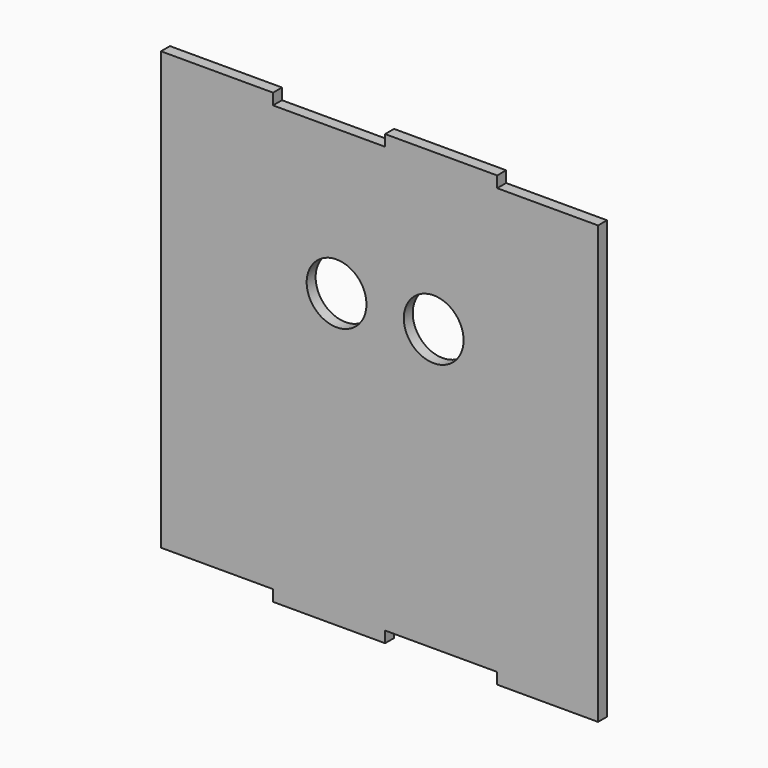
from build123d import *

# Parameters (mm, degrees)
F0_R     = 8
F1_DEPTH = 1.5


# Not quite as in the source:
# - a feature names something its author has since deleted; it is built from what else it names


with BuildPart() as f1:
    # F0 (on Front) → F1 (new body, symmetric)
    with BuildSketch(Plane.XZ):
        Polygon((-30, -2.9994321861), (0, -2.9994321861), (0, 0), (30, 0), (30, -2.9994321861), (57, -2.9994321861), (57, 114.0005678139), (30, 114.0005678139), (30, 117.0005678139), (0, 117.0005678139), (0, 114.0005678139), (-30, 114.0005678139), (-30, 117.0005678139), (-60, 117.0005678139), (-60, 0), (-30, 0), align=None)
        with Locations((-13, 75.2281695604)):
            Circle(F0_R, mode=Mode.SUBTRACT)
        with Locations((13, 75.2218647463)):
            Circle(F0_R, mode=Mode.SUBTRACT)
    extrude(amount=F1_DEPTH, both=True)


solid = f1.part
